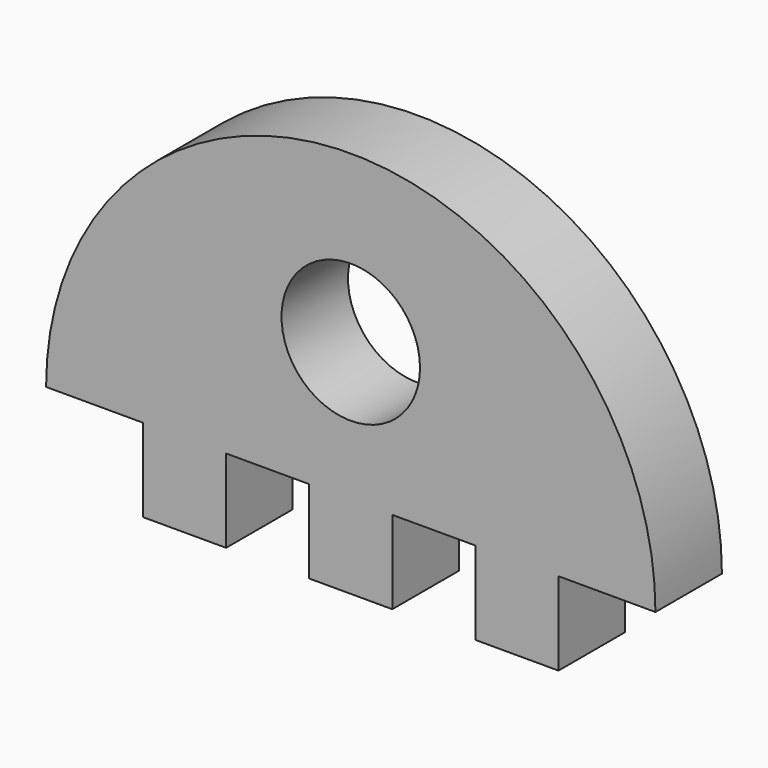
from build123d import *

# Parameters (mm, degrees)
F0_R     = 2.5
F1_DEPTH = 3


# Not quite as in the source:
# - a feature names something its author has since deleted; it is built from what else it names


with BuildPart() as f1:
    # F0 (on Front) → F1 (new body)
    with BuildSketch(Plane.XZ):
        with BuildLine():
            Line((7.5, 0), (11, 0))
            ThreePointArc((11, 0), (0, 11), (-11, 0))
            Line((-11, 0), (-7.5, 0))
            Line((-7.5, 0), (-7.5, -3))
            Line((-7.5, -3), (-4.5, -3))
            Line((-4.5, -3), (-4.5, 0))
            Line((-4.5, 0), (-1.5, 0))
            Line((-1.5, 0), (-1.5, -3))
            Line((-1.5, -3), (1.5, -3))
            Line((1.5, -3), (1.5, 0))
            Line((1.5, 0), (4.5, 0))
            Line((4.5, 0), (4.5, -3))
            Line((4.5, -3), (7.5, -3))
            Line((7.5, -3), (7.5, 0))
        make_face()
        with Locations((0, 5)):
            Circle(F0_R, mode=Mode.SUBTRACT)
    extrude(amount=F1_DEPTH)


solid = f1.part
